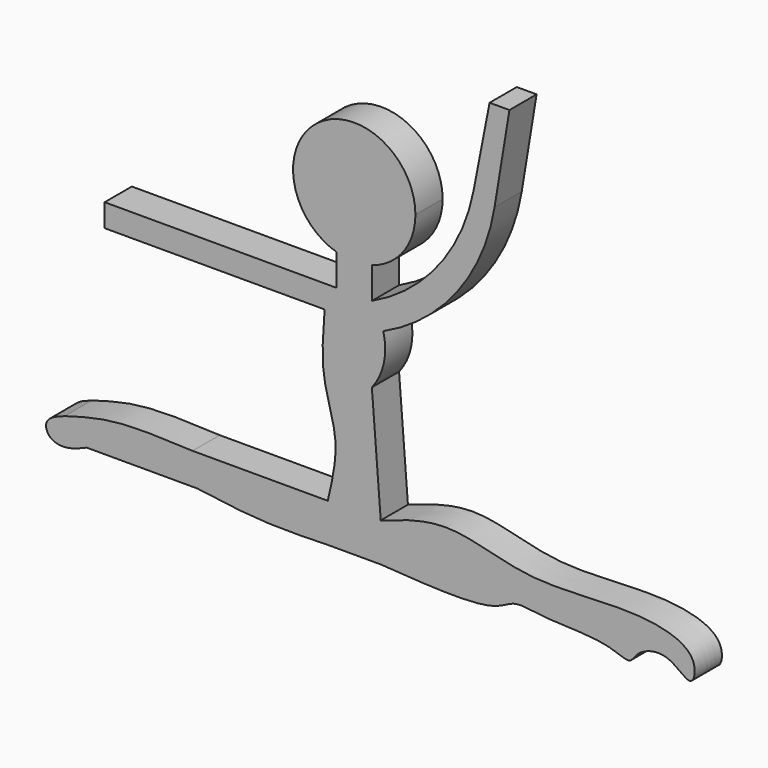
from build123d import *

# Parameters (mm, degrees)
F1_DEPTH = 6.35


# Not quite as in the source:
# - a feature names something its author has since deleted; it is built from what else it names


with BuildPart() as f1:
    # F0 (on Front) → F1 (new body)
    with BuildSketch(Plane.XZ):
        with BuildLine():
            ThreePointArc((3.2900583662, 10.1591339407), (9.1719754449, 14.2848451287), (11.43, 21.1053851687))
            ThreePointArc((11.43, 21.1053851687), (-6.82054004, 30.2773606136), (-3.2900583662, 10.1591339407))
            ThreePointArc((-3.2900583662, 10.1591339407), (0, 9.6753851687), (3.2900583662, 10.1591339407))
        make_face()
        with BuildLine():
            ThreePointArc((3.2900583662, 10.1591339407), (0, 9.6753851687), (-3.2900583662, 10.1591339407))
            Line((-3.2900583662, 10.1591339407), (-3.2900583662, 4.2767086129))
            Line((-3.2900583662, 4.2767086129), (-46.6294512153, 4.2767086129))
            Line((-46.6294512153, 4.2767086129), (-46.6294512153, 0))
            Line((-46.6294512153, 0), (-5.5364955777, 0))
            add(Edge.make_bspline(
                [(-5.5364955777, 0), (-5.846473931, -3.9091577352), (-6.441928195, -11.4184712635), (-2.4753350411, -20.717984445), (-4.1131079796, -27.7055383728), (-4.950948954, -31.2801846833)],
                knots=[0, 0, 0, 0, 0.3465540249, 0.6657144591, 1, 1, 1, 1], degree=3))
            Line((-4.950948954, -31.2801846833), (-30.2072484046, -31.2801846833))
            add(Edge.make_bspline(
                [(-30.2072484046, -31.2801846833), (-35.4185782709, -31.0411958162), (-44.7939905391, -30.6112443041), (-51.2490391451, -32.5017979902), (-54.1160441935, -33.341486007)],
                knots=[0, 0, 0, 0, 0.5558507421, 1, 1, 1, 1], degree=3))
            add(Edge.make_bspline(
                [(-54.1160441935, -33.341486007), (-55.5286452206, -33.854603905), (-58.0351409859, -34.7650717679), (-57.3014191928, -37.9783158116), (-53.9282463564, -38.8392803933), (-51.3814983639, -37.7688277416), (-49.9947071075, -37.1859297156)],
                knots=[0, 0, 0, 0, 0.2683530976, 0.4761612725, 0.7147519232, 1, 1, 1, 1], degree=3))
            Line((-49.9947071075, -37.1859297156), (-29.329361394, -37.1859297156))
            add(Edge.make_bspline(
                [(-29.329361394, -37.1859297156), (-25.3198216255, -37.7475429691), (-17.2732489539, -38.874620419), (-9.0677276948, -38.6482800707), (-4.950948954, -38.5347232223)],
                knots=[0, 0, 0, 0, 0.4982916245, 1, 1, 1, 1], degree=3))
            Line((-4.950948954, -38.5347232223), (4.950948954, -38.5347232223))
            add(Edge.make_bspline(
                [(4.950948954, -31.2801846833), (9.1079723115, -29.8139525042), (17.7937353891, -26.7503793103), (32.6902038965, -32.9435441408), (51.3912064132, -30.1338297579), (64.4437974876, -33.2099452487), (63.3035332188, -40.8742099619), (58.6772356204, -35.1370782722), (52.8158624781, -36.975462438), (51.6362128477, -40.0721494762), (47.146816139, -37.3115873926), (35.4532116414, -37.6125697148), (29.8372100476, -36.1641615463), (25.7253514724, -39.9381489762), (13.4111881556, -39.1062591579), (4.950948954, -38.5347232223)],
                knots=[0, 0, 0, 0, 0.0949511611, 0.1983927484, 0.3158351085, 0.4050526471, 0.4558672869, 0.5146179799, 0.5763072953, 0.6169649042, 0.670738832, 0.762635828, 0.8238542417, 0.8789820135, 1, 1, 1, 1], degree=3))
            Line((4.950948954, -31.2801846833), (3.2900583662, -9.9441846833))
            ThreePointArc((3.2900583662, -9.9441846833), (5.5325425162, -5.2243959207), (5.4284829638, 0))
            ThreePointArc((5.4284829638, 0), (4.5867025548, 2.2530665196), (3.2900583662, 4.2788051125))
            Line((3.2900583662, 4.2788051125), (3.2900583662, 10.1591339407))
        make_face()
        with BuildLine():
            ThreePointArc((22.2743526101, 28.5083446652), (15.6945827163, 14.1116732403), (3.2900583662, 4.2788051125))
            ThreePointArc((3.2900583662, 4.2788051125), (4.5867025548, 2.2530665196), (5.4284829638, 0))
            ThreePointArc((5.4284829638, 0), (19.2171447998, 10.9559029), (26.2115225196, 27.1187517792))
            Line((26.2115225196, 27.1187517792), (28.9907027036, 44.0254285932))
            Line((28.9907027036, 44.0254285932), (25.2851303667, 44.0254285932))
            add(Edge.make_bspline(
                [(22.2743526101, 28.5083446652), (23.2779451956, 33.6807059745), (24.2815377812, 38.8530672838), (25.2851303667, 44.0254285932)],
                knots=[0, 0, 0, 0, 15.8064757719, 15.8064757719, 15.8064757719, 15.8064757719], degree=3))
        make_face()
    extrude(amount=F1_DEPTH)


solid = f1.part
